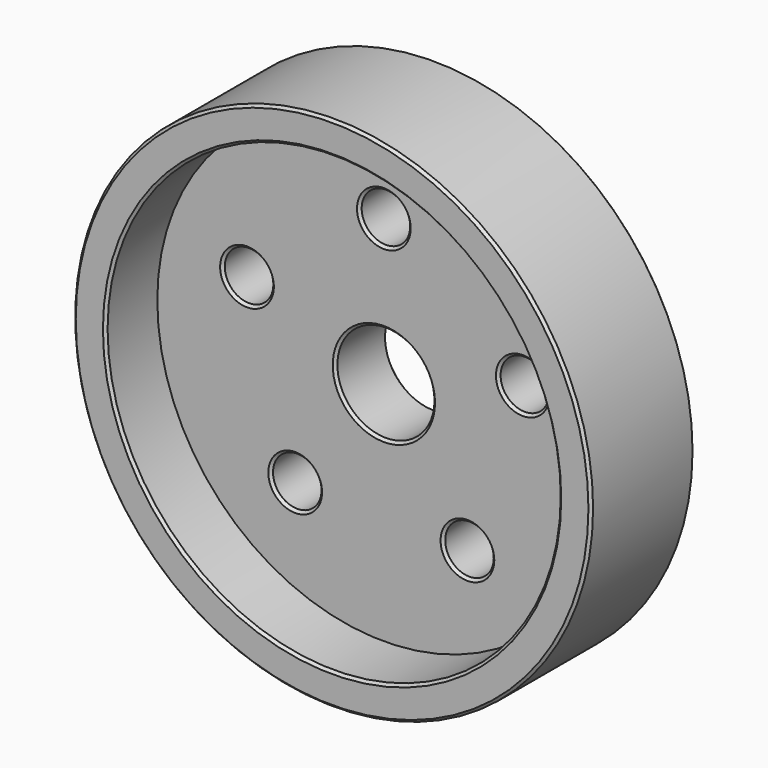
from build123d import *

# Parameters (mm, degrees)
F0_R     = 50.8
F0_R_2   = 9.525
F1_DEPTH = 25.4
F2_R     = 44.45
F2_R_2   = 9.525
F3_DEPTH = 12.7
F4_R     = 4.7625
F5_DEPTH = 12.701
F6_SIZE  = 0.508


with BuildPart() as f1:
    # F0 (on Front) → F1 (new body)
    with BuildSketch(Plane.XZ):
        Circle(F0_R)
        Circle(F0_R_2, mode=Mode.SUBTRACT)
    extrude(amount=F1_DEPTH)

    # F2 (on face) → F3 (cut)
    with BuildSketch(Plane.XZ.offset(25.4)):
        Circle(F2_R)
        Circle(F2_R_2, mode=Mode.SUBTRACT)
    extrude(amount=-F3_DEPTH, mode=Mode.SUBTRACT)

    # F4 (on face) → F5 (cut, through all)
    with BuildSketch(Plane.XZ.offset(12.7)):
        with Locations((-26.851716639, 9.7732255955)):
            Circle(F4_R)
        with Locations((0, 28.575)):
            Circle(F4_R)
        with Locations((27.2524618676, 8.5926682208)):
            Circle(F4_R)
        with Locations((16.3899466687, -23.4072696656)):
            Circle(F4_R)
        with Locations((-17.3953578339, -22.6700716988)):
            Circle(F4_R)
    extrude(amount=-F5_DEPTH, mode=Mode.SUBTRACT)

    # F6
    f6_edges = [f1.edges().sort_by_distance(p)[0] for p in [
        (-44.45, -25.4, 0),
        (-4.7625, -12.7, 28.575),
        (-31.614217, -12.7, 9.773226),
        (-9.525, -12.7, 0),
        (-22.157858, -12.7, -22.670072),
        (-50.8, 0, 0),
        (11.627447, -12.7, -23.40727),
        (22.489962, -12.7, 8.592668),
        (-50.8, -25.4, 0),
        (-4.7625, 0, 28.575),
        (-31.614217, 0, 9.773226),
        (-22.157858, 0, -22.670072),
        (11.627447, 0, -23.40727),
        (22.489962, 0, 8.592668),
        (-9.525, 0, 0),
    ]]
    chamfer(f6_edges, length=F6_SIZE)


solid = f1.part
